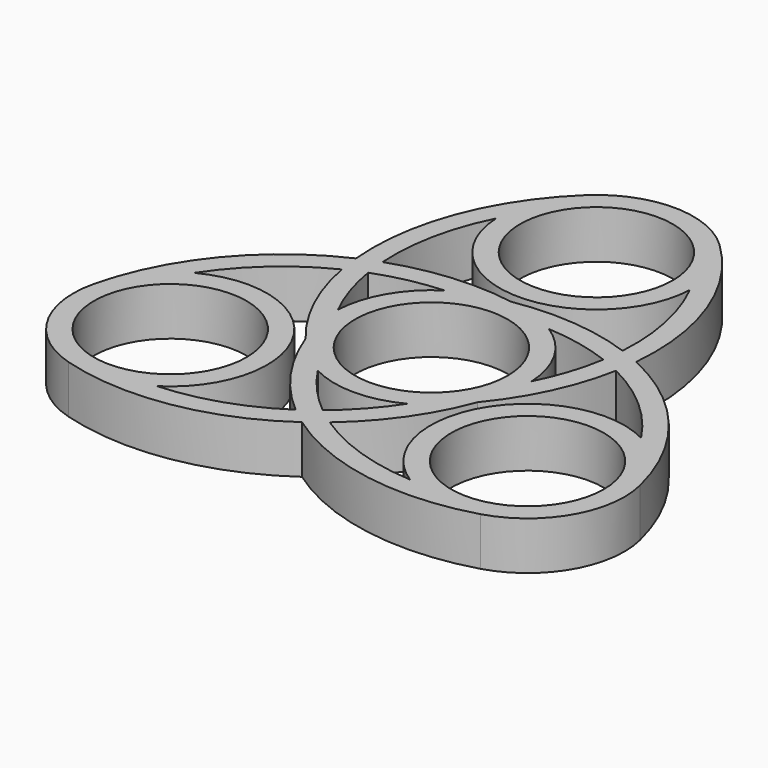
from build123d import *

# Parameters (mm, degrees)
F0_R            = 11.1
F1_DEPTH        = 7
F1_COPIES_COUNT = 3


# Not quite as in the source:
# - a pattern or mirror of a feature is missing from the dataset's text; its kind, count and spacing are read off the source's solid


with BuildPart() as f1:
    # F0 (on Top) → F1 (new body)
    with BuildSketch(Plane.XY):
        with BuildLine():
            ThreePointArc((14.0864100033, 29.3810870676), (14.0966020914, 29.690468941), (14.1, 30))
            ThreePointArc((14.1, 30), (12.9626271297, 35.5479994499), (9.7340002984, 40.200943005))
            ThreePointArc((9.7340002984, 40.200943005), (0, 44.1), (-9.7340002984, 40.200943005))
            ThreePointArc((-9.7340002984, 40.200943005), (-13.0812960888, 35.2620996416), (-14.0864100033, 29.3810870676))
            ThreePointArc((-14.0864100033, 29.3810870676), (0, 15.9), (14.0864100033, 29.3810870676))
        make_face()
        with Locations((0, 30)):
            Circle(F0_R, mode=Mode.SUBTRACT)
        with BuildLine():
            ThreePointArc((9.7340002984, 40.200943005), (12.9626271297, 35.5479994499), (14.1, 30))
            ThreePointArc((14.1, 30), (14.0966020914, 29.690468941), (14.0864100033, 29.3810870676))
            ThreePointArc((14.0864100033, 29.3810870676), (17.5199942586, 15), (14.0864100033, 0.6189129324))
            ThreePointArc((14.0864100033, 0.6189129324), (14.0966020914, 0.309531059), (14.1, 0))
            ThreePointArc((14.1, 0), (12.9626271297, -5.5479994499), (9.7340002984, -10.200943005))
            ThreePointArc((9.7340002984, -10.200943005), (20.5199942586, 15), (9.7340002984, 40.200943005))
        make_face()
        with BuildLine():
            ThreePointArc((-9.7340002984, -10.200943005), (0, -14.1), (9.7340002984, -10.200943005))
            ThreePointArc((9.7340002984, -10.200943005), (12.9626271297, -5.5479994499), (14.1, 0))
            ThreePointArc((14.1, 0), (14.0966020914, 0.309531059), (14.0864100033, 0.6189129324))
            ThreePointArc((14.0864100033, 0.6189129324), (0, 14.1), (-14.0864100033, 0.6189129324))
            ThreePointArc((-14.0864100033, 0.6189129324), (-13.0812960888, -5.2620996416), (-9.7340002984, -10.200943005))
        make_face()
        Circle(F0_R, mode=Mode.SUBTRACT)
        with BuildLine():
            ThreePointArc((-14.0864100033, 29.3810870676), (-13.0812960888, 35.2620996416), (-9.7340002984, 40.200943005))
            ThreePointArc((-9.7340002984, 40.200943005), (-20.5199942586, 15), (-9.7340002984, -10.200943005))
            ThreePointArc((-9.7340002984, -10.200943005), (-13.0812960888, -5.2620996416), (-14.0864100033, 0.6189129324))
            ThreePointArc((-14.0864100033, 0.6189129324), (-17.5199942586, 15), (-14.0864100033, 29.3810870676))
        make_face()
    extrude(amount=F1_DEPTH)

    # F1_copies: F1 ×3 about axis
    f1_copies_axis = Axis((0, 0, 0), (0, 0, 1))


with BuildPart() as f1_1:
    add(f1.part)
    for i in range(1, F1_COPIES_COUNT):
        add(f1.part.rotate(f1_copies_axis, i * 360 / F1_COPIES_COUNT))


solid = f1_1.part
